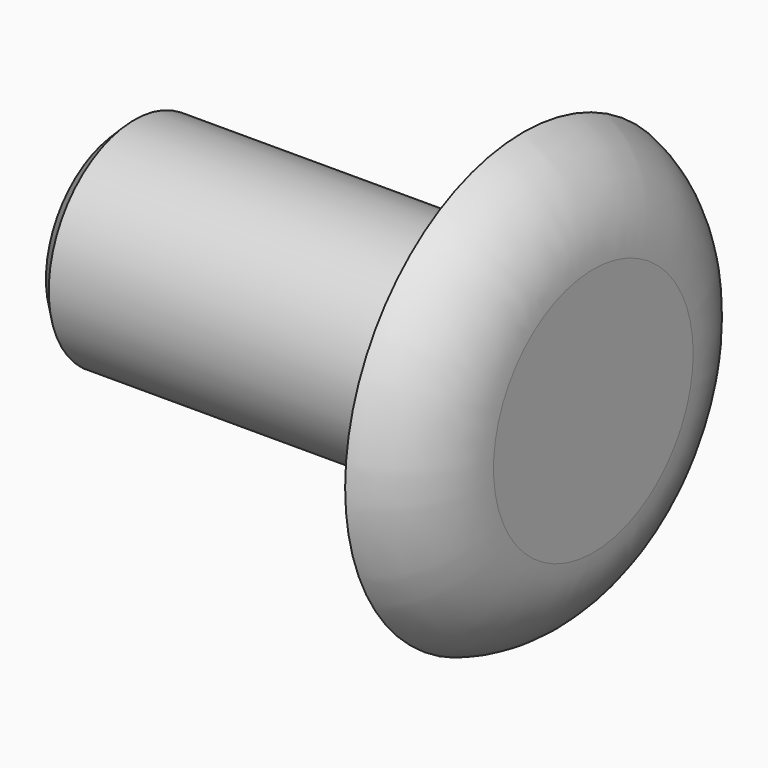
from build123d import *

# Parameters (mm, degrees)
F6_R           = 2.286
F8_DEPTH       = 9.35
F9_SIZE        = 0.3
F10_R          = 4.7503425206
F11_DEPTH      = 0.75
F11_DEPTH_BACK = 0.75


# Not quite as in the source:
# - a fillet or chamfer that OpenCascade refuses, or shapes differently, is made with other operations: its cross-section is extruded or revolved along the edge and cut away or added
# - the program builds the solid bodies; features that only make, move or delete a surface that nothing else refers to are left out


with BuildPart() as f8:
    # F6 (on Right) → F8 (new body)
    with BuildSketch(Plane.YZ):
        Circle(F6_R)
    extrude(amount=-F8_DEPTH)

    # F9
    f9_edges = [f8.edges().sort_by_distance(p)[0] for p in [
        (-9.35, -2.286, 0),
    ]]
    chamfer(f9_edges, length=F9_SIZE)

    # F10 (on Right) → F11 (join, two sides)
    with BuildSketch(Plane.YZ) as f11_sk:
        Circle(F10_R)
    extrude(amount=F11_DEPTH)
    extrude(f11_sk.sketch, amount=-F11_DEPTH_BACK)

    # F12: fillet of radius 2.2 on 1 edges, made by hand

    # F12_s1 → F12_t2 (revolve, cut)
    with BuildSketch(Plane.XY):
        with BuildLine():
            ThreePointArc((-0.75, 4.7503425206), (0.3360571099, 3.949200417), (0.75, 2.6646771591))
            Line((0.75, 2.6646771591), (0.75, 4.7503425206))
            Line((0.75, 4.7503425206), (-0.75, 4.7503425206))
        make_face()
    revolve(axis=Axis((0.75, 0, 0), (1, 0, 0)), mode=Mode.SUBTRACT)


solid = f8.part
